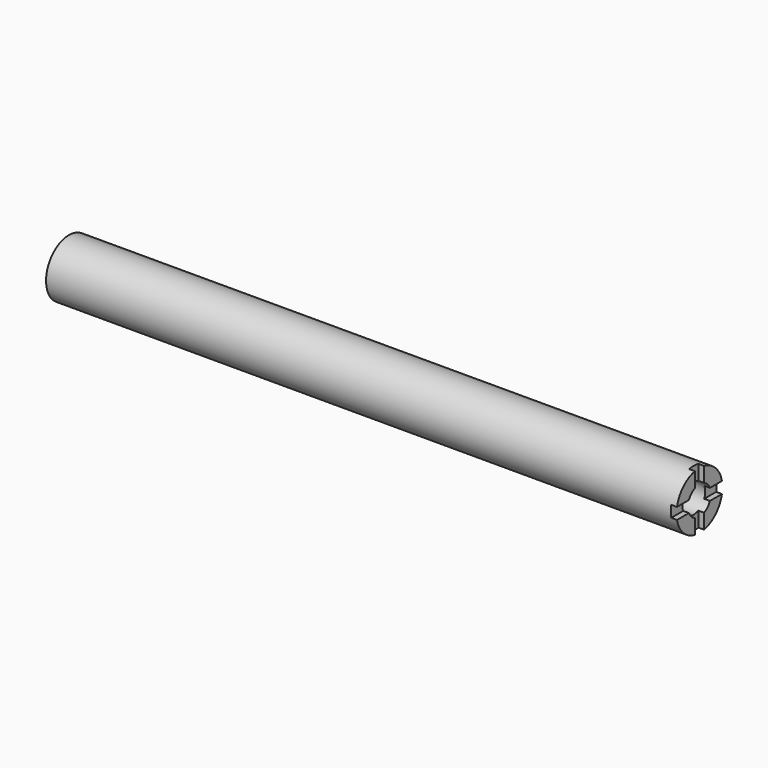
from build123d import *

# Parameters (mm, degrees)
F0_R            = 12.7
F1_DEPTH        = 279.4
F2_R            = 6.35
F3_DEPTH        = 25.4
F5_DEPTH        = 2.54
F5_COPIES_COUNT = 4


# Not quite as in the source:
# - a pattern or mirror of a feature is missing from the dataset's text; its kind, count and spacing are read off the source's solid
# - a feature names something its author has since deleted; it is built from what else it names


with BuildPart() as f1:
    # F0 (on Right) → F1 (new body)
    with BuildSketch(Plane.YZ):
        Circle(F0_R)
    extrude(amount=-F1_DEPTH)

    # F2 (on face) → F3 (cut)
    with BuildSketch(Plane.YZ):
        Circle(F2_R)
    extrude(amount=-F3_DEPTH, mode=Mode.SUBTRACT)

    # F4 (on face) → F5 (cut)
    with BuildSketch(Plane.YZ):
        with BuildLine():
            ThreePointArc((-5.8198711326, -2.54), (-6.35, 0), (-5.8198711326, 2.54))
            Line((-5.8198711326, 2.54), (-12.4434078933, 2.54))
            ThreePointArc((-12.4434078933, 2.54), (-12.7, 0), (-12.4434078933, -2.54))
            Line((-12.4434078933, -2.54), (-5.8198711326, -2.54))
        make_face()
    f5 = extrude(amount=-F5_DEPTH, mode=Mode.SUBTRACT)

    # F5_copies: F5 ×4 about axis
    f5_copies_axis = Axis((0, 0, 0), (1, 0, 0))
    for i in range(1, F5_COPIES_COUNT):
        add(f5.rotate(f5_copies_axis, i * 360 / F5_COPIES_COUNT), mode=Mode.SUBTRACT)


solid = f1.part
